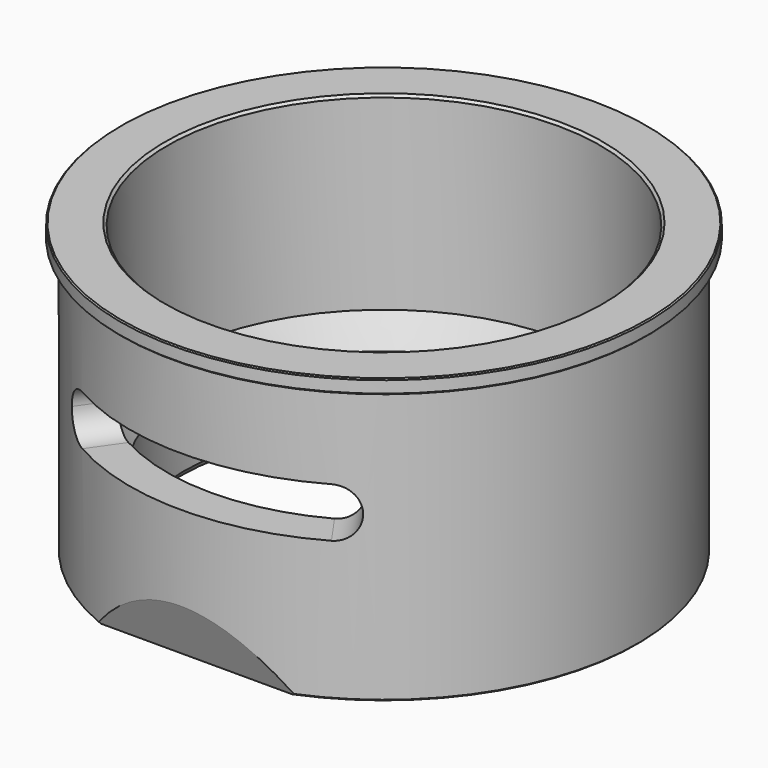
from build123d import *

# Parameters (mm, degrees)
F2_R          = 0.381
F3_SIZE       = 0.381
F4_SIZE       = 0.7874
F5_SIZE2      = 0.9092112039
F5_SIZE       = 1.5748
F7_DEPTH      = 84.1385
F7_DEPTH_BACK = 84.1385
F8_SIZE       = 0.381
F11_DEPTH     = 15.875
F12_R         = 7.9375
F13_R         = 7.93749


# Not quite as in the source:
# - a fillet or chamfer is up to 0.001 mm smaller than in the source, because OpenCascade refuses the exact size


with BuildPart() as f1:
    # F0 (on Right) → F1 (revolve)
    with BuildSketch(Plane.YZ):
        Polygon((84.1375, -4.5212), (84.1375, 0), (69.0626, 0), (69.0626, -60.325), (63.8937, -69.2777974192), (63.8937, -92.075), (80.9625, -92.075), (80.9625, -4.5212), align=None)
    revolve(axis=Axis((0, 0, -46.0375), (0, 0, -1)))

    # F2
    f2_edges = [f1.edges().sort_by_distance(p)[0] for p in [
        (0, -80.9625, -4.5212),
    ]]
    fillet(f2_edges, radius=F2_R)

    # F3
    f3_edges = [f1.edges().sort_by_distance(p)[0] for p in [
        (0, -84.1375, -4.5212),
        (0, -84.1375, 0),
        (0, 84.1375, -2.2606),
    ]]
    chamfer(f3_edges, length=F3_SIZE)

    # F4
    f4_edges = [f1.edges().sort_by_distance(p)[0] for p in [
        (0, -69.0626, 0),
    ]]
    chamfer(f4_edges, length=F4_SIZE)

    # F5
    f5_edges = [f1.edges().sort_by_distance(p)[0] for p in [
        (0, -63.8937, -92.075),
    ]]
    chamfer(f5_edges, length=F5_SIZE, length2=F5_SIZE2)

    # F6 (on Right) → F7 (cut, two sides)
    with BuildSketch(Plane.YZ) as f7_sk:
        Polygon((-80.9625, -74.6285183865), (-80.9625, -92.075), (-74.6125, -92.075), align=None)
    extrude(amount=F7_DEPTH, mode=Mode.SUBTRACT)
    extrude(f7_sk.sketch, amount=-F7_DEPTH_BACK, mode=Mode.SUBTRACT)

    # F8
    f8_edges = [f1.edges().sort_by_distance(p)[0] for p in [
        (79.359123, 16.032964, -92.075),
    ]]
    chamfer(f8_edges, length=F8_SIZE)

    # F10 (on offset) → F11 (cut)
    with BuildSketch(Plane.XY.offset(-31.75)):
        with BuildLine():
            Line((-39.6126799931, -56.5727699739), (-46.4381822281, -66.3205973857))
            ThreePointArc((-46.4381822281, -66.3205973857), (0, -80.9625), (46.4381822281, -66.3205973857))
            Line((46.4381822281, -66.3205973857), (39.6126799931, -56.5727699739))
            ThreePointArc((39.6126799931, -56.5727699739), (0, -69.0626), (-39.6126799931, -56.5727699739))
        make_face()
    extrude(amount=-F11_DEPTH, mode=Mode.SUBTRACT)

    # F12
    f12_edges = [f1.edges().sort_by_distance(p)[0] for p in [
        (-43.025431, -61.446684, -31.75),
        (43.025431, -61.446684, -31.75),
    ]]
    fillet(f12_edges, radius=F12_R)

    # F13 (radius 7.9375 in the source; OpenCascade refuses exactly that, so slightly less here)
    f13_edges = [f1.edges().sort_by_distance(p)[0] for p in [
        (-43.025431, -61.446684, -47.625),
        (43.025431, -61.446684, -47.625),
    ]]
    fillet(f13_edges, radius=F13_R)


solid = f1.part
